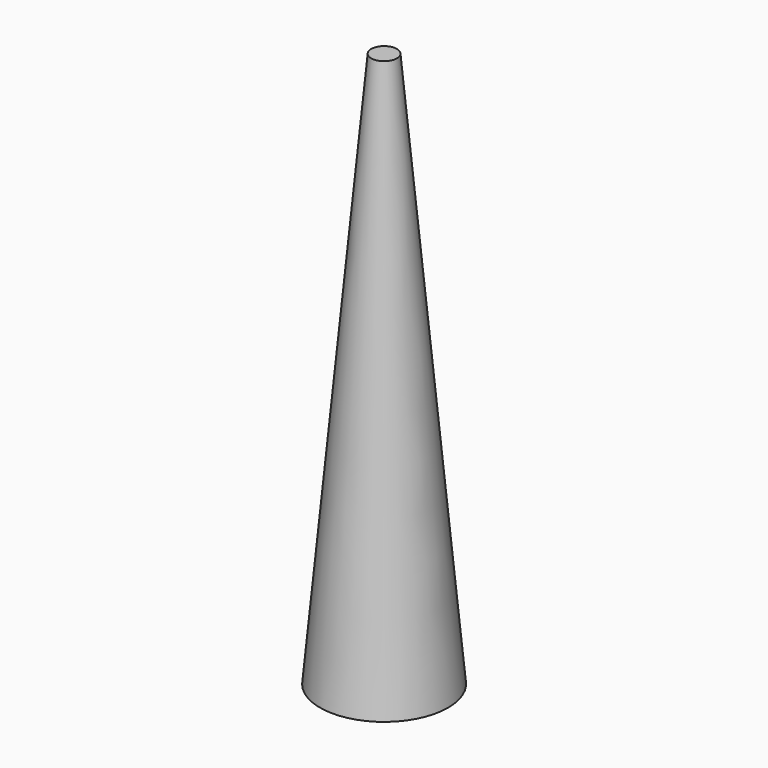
from build123d import *

# Parameters (mm, degrees)
F0_R     = 15
F1_DEPTH = 130
F2_SIZE2 = 129.99999
F2_SIZE  = 11.99999


# Not quite as in the source:
# - a fillet or chamfer is up to 0.001 mm smaller than in the source, because OpenCascade refuses the exact size


with BuildPart() as f1:
    # F0 (on Top) → F1 (new body)
    with BuildSketch(Plane.XY):
        Circle(F0_R)
    extrude(amount=F1_DEPTH)

    # F2 (size 12 and 130 in the source; OpenCascade refuses exactly that, so slightly less here)
    f2_edges = [f1.edges().sort_by_distance(p)[0] for p in [
        (-15, 0, 130),
    ]]
    f2_side = f1.faces().sort_by_distance((0, 0, 130))[0]
    chamfer(f2_edges, length=F2_SIZE, length2=F2_SIZE2, reference=f2_side)


solid = f1.part
